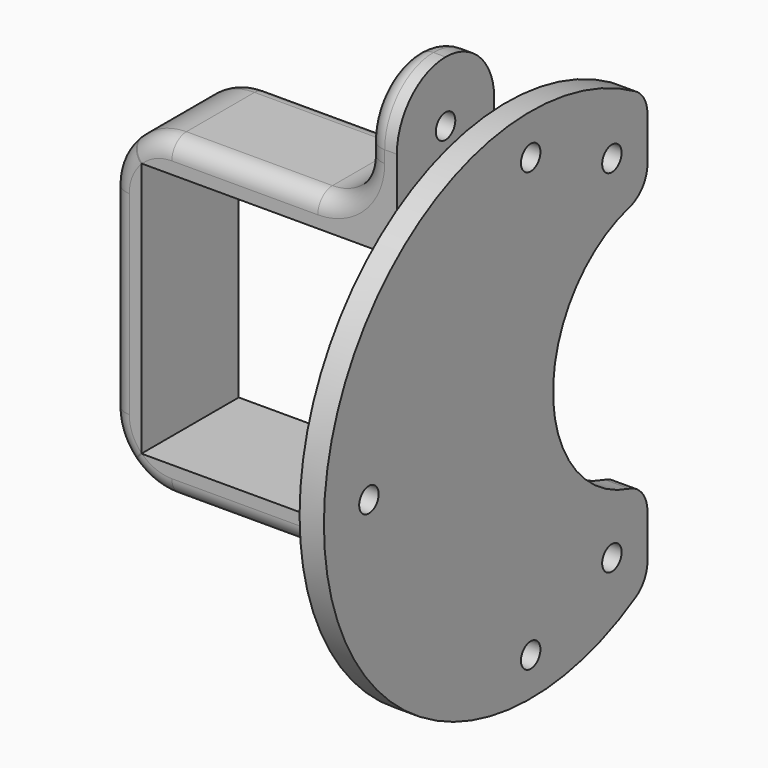
from build123d import *

# Parameters (mm, degrees)
F1_DEPTH    = 20
F2_R        = 8
F3_R        = 9.99999
F4_R        = 3
F7_R        = 2
F8_DEPTH    = 4
F9_D        = 4
F9_ON_F5_D  = 4
F10_D       = 4
F10_ON_F5_D = 4


# Not quite as in the source:
# - a fillet or chamfer is up to 0.001 mm smaller than in the source, because OpenCascade refuses the exact size


with BuildPart() as f1:
    # F0 (on Front) → F1 (new body)
    with BuildSketch(Plane.XZ):
        Polygon((-52, 21), (-10, 21), (-10, 46), (-15, 46), (-15, 26), (-57, 26), (-57, -26), (-15, -26), (-15, -46), (-10, -46), (-10, -21), (-52, -21), align=None)
    extrude(amount=F1_DEPTH)

    # F2
    f2_edges = [f1.edges().sort_by_distance(p)[0] for p in [
        (-15, -10, -26),
        (-15, -10, 26),
    ]]
    fillet(f2_edges, radius=F2_R)

    # F3 (radius 10 in the source; OpenCascade refuses exactly that, so slightly less here)
    f3_edges = [f1.edges().sort_by_distance(p)[0] for p in [
        (-12.5, 0, 46),
        (-12.5, -20, 46),
        (-12.5, 0, -46),
        (-12.5, -20, -46),
        (-57, -10, -26),
        (-57, -10, 26),
    ]]
    fillet(f3_edges, radius=F3_R)

    # F4
    f4_edges = [f1.edges().sort_by_distance(p)[0] for p in [
        (-57, 0, 0),
    ]]
    fillet(f4_edges, radius=F4_R)

    # F9 (through all)
    with Locations(Plane.YZ.offset(-10)):
        with Locations((-10, -36)):
            Hole(F9_D / 2)

    # F9 on F5 (through all)
    with Locations(Plane.YZ.offset(-10)):
        with Locations((-10, 36)):
            Hole(F9_ON_F5_D / 2)


with BuildPart() as f8:
    # F7 (on Right) → F8 (new body)
    with BuildSketch(Plane.YZ):
        with BuildLine():
            ThreePointArc((14, 32.5194938452), (13.3397388554, 35.0027712494), (11.5333333333, 36.8302040212))
            ThreePointArc((11.5333333333, 36.8302040212), (-52.5, 0.1891675245), (11.5333333333, -36.4518689722))
            ThreePointArc((11.5333333333, -36.4518689722), (13.3397388554, -34.6244362004), (14, -32.1411587962))
            Line((14, -32.1411587962), (14, -25.009258036))
            ThreePointArc((14, -25.009258036), (12.9621576699, -21.9594536818), (10.2794773604, -20.1757357505))
            ThreePointArc((10.2794773604, -20.1757357505), (-5.3960650728, 0.1891675245), (10.2794773604, 20.5540707995))
            ThreePointArc((10.2794773604, 20.5540707995), (12.9621576699, 22.3377887308), (14, 25.387593085))
            Line((14, 25.387593085), (14, 32.5194938452))
        make_face()
        with Locations((-43.2497895028, 0)):
            Circle(F7_R, mode=Mode.SUBTRACT)
        with Locations((6.6871778265, -28.7138723059)):
            Circle(F7_R, mode=Mode.SUBTRACT)
        with Locations((6.6871778265, 29.0922073549)):
            Circle(F7_R, mode=Mode.SUBTRACT)
    extrude(amount=F8_DEPTH)

    # F10 (through all)
    with Locations(Plane(origin=(-10, 0, 0), x_dir=(0, 1, 0), z_dir=(-1, 0, 0))):
        with Locations((-10, 36)):
            Hole(F10_D / 2)

    # F10 on F5 (through all)
    with Locations(Plane(origin=(-10, 0, 0), x_dir=(0, 1, 0), z_dir=(-1, 0, 0))):
        with Locations((-10, -36)):
            Hole(F10_ON_F5_D / 2)


solid = Compound([f1.part, f8.part])
